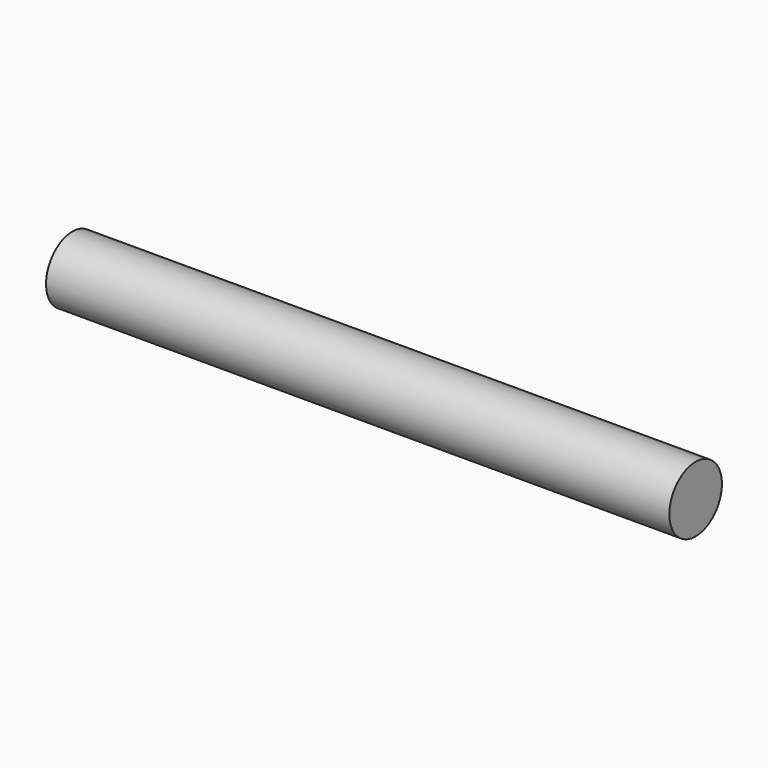
from build123d import *

# Parameters (mm, degrees)
F0_R     = 3.683
F1_DEPTH = 69.85


# Not quite as in the source:
# - the program builds the solid bodies; features that only make, move or delete a surface that nothing else refers to are left out


with BuildPart() as f1:
    # F0 (on Right) → F1 (new body)
    with BuildSketch(Plane.YZ):
        with Locations((-26.563832688, 32.5135998428)):
            Circle(F0_R)
    extrude(amount=F1_DEPTH)


solid = f1.part
